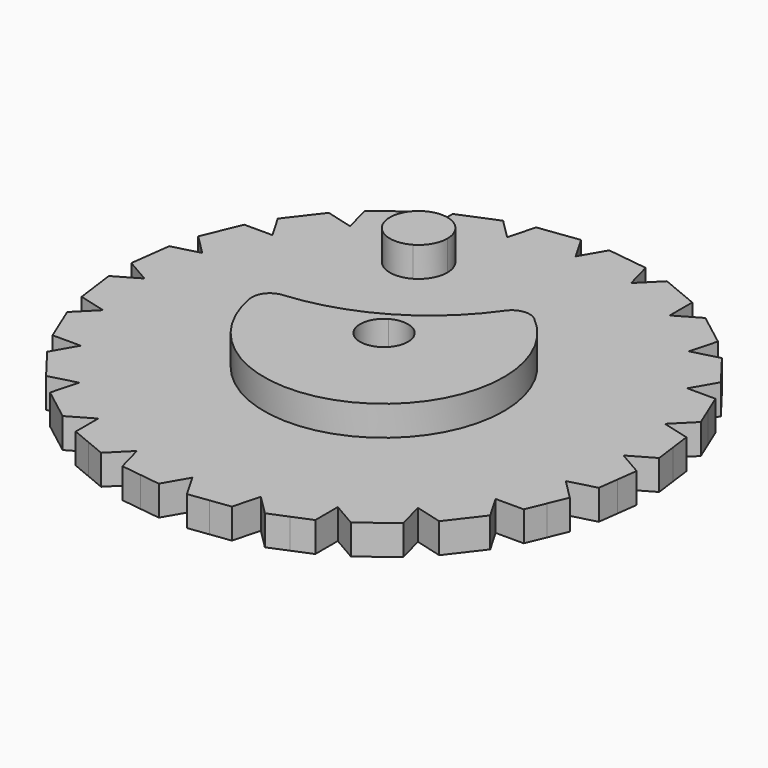
from build123d import *

# Parameters (mm, degrees)
F0_R     = 20
F2_DEPTH = 2.5
F3_DEPTH = 5
F4_DEPTH = 2.5
F5_R     = 1.5


with BuildPart() as f2:
    # F0 (on Top) → F2 (new body)
    with BuildSketch(Plane.XY):
        with Locations((30, 0)):
            Circle(F0_R)
        with BuildLine():
            ThreePointArc((20, 0), (24.4828773608, 0.5901820009), (28.6602540378, 2.3205080757))
            ThreePointArc((28.6602540378, 2.3205080757), (32.2474487139, 5.0730593618), (35, 8.6602540378))
            ThreePointArc((35, 8.6602540378), (35, -8.6602540378), (20, 0))
        make_face(mode=Mode.SUBTRACT)
        with BuildLine():
            ThreePointArc((24.9, 12.9903810568), (24.5784609691, 11.7903810568), (23.7, 10.9119200877))
            ThreePointArc((23.7, 10.9119200877), (20.4215390309, 14.1903810568), (24.9, 12.9903810568))
        make_face(mode=Mode.SUBTRACT)
    extrude(amount=F2_DEPTH)

    # F0 (on Top) → F3 (join)
    with BuildSketch(Plane.XY):
        with BuildLine():
            ThreePointArc((24.9, 12.9903810568), (20.4215390309, 14.1903810568), (23.7, 10.9119200877))
            ThreePointArc((23.7, 10.9119200877), (24.5784609691, 11.7903810568), (24.9, 12.9903810568))
        make_face()
        with BuildLine():
            ThreePointArc((35, 8.6602540378), (32.2474487139, 5.0730593618), (28.6602540378, 2.3205080757))
            ThreePointArc((28.6602540378, 2.3205080757), (24.4828773608, 0.5901820009), (20, 0))
            ThreePointArc((20, 0), (35, -8.6602540378), (35, 8.6602540378))
        make_face()
        with BuildLine():
            ThreePointArc((32, 0), (29, -1.7320508076), (29, 1.7320508076))
            ThreePointArc((29, 1.7320508076), (31, 1.7320508076), (32, 0))
        make_face(mode=Mode.SUBTRACT)
    extrude(amount=F3_DEPTH)

    # F1 (on Top) → F4 (join)
    with BuildSketch(Plane.XY):
        with BuildLine():
            Line((31.1749923535, 22.0351464548), (30, 20))
            ThreePointArc((30, 20), (32.6105238444, 19.8288972275), (35.1763809021, 19.3185165258))
            Line((35.1763809021, 19.3185165258), (34.5681601042, 21.5884274457))
            Line((34.5681601042, 21.5884274457), (32.8715762288, 21.8117869502))
            Line((32.8715762288, 21.8117869502), (31.1749923535, 22.0351464548))
        make_face()
        with BuildLine():
            Line((7.9648535452, 1.1749923535), (10, 0))
            Line((10, 0), (7.9648535452, -1.1749923535))
            Line((7.9648535452, -1.1749923535), (8.1882130498, -2.8715762288))
            Line((8.1882130498, -2.8715762288), (8.4115725543, -4.5681601042))
            Line((8.4115725543, -4.5681601042), (10.6814834742, -5.1763809021))
            Line((10.6814834742, -5.1763809021), (9.0197933522, -6.8380710241))
            Line((9.0197933522, -6.8380710241), (9.6746502848, -8.419035512))
            Line((9.6746502848, -8.419035512), (10.3295072173, -10))
            Line((10.3295072173, -10), (12.6794919243, -10))
            Line((12.6794919243, -10), (11.5044995708, -12.0351464548))
            Line((11.5044995708, -12.0351464548), (12.5462265136, -13.3927514382))
            Line((12.5462265136, -13.3927514382), (13.5879534564, -14.7503564216))
            Line((13.5879534564, -14.7503564216), (15.8578643763, -14.1421356237))
            Line((15.8578643763, -14.1421356237), (15.2496435784, -16.4120465436))
            Line((15.2496435784, -16.4120465436), (16.6072485618, -17.4537734864))
            Line((16.6072485618, -17.4537734864), (17.9648535452, -18.4955004292))
            Line((17.9648535452, -18.4955004292), (20, -17.3205080757))
            Line((20, -17.3205080757), (20, -19.6704927827))
            Line((20, -19.6704927827), (21.580964488, -20.3253497152))
            Line((21.580964488, -20.3253497152), (23.1619289759, -20.9802066478))
            Line((23.1619289759, -20.9802066478), (24.8236190979, -19.3185165258))
            Line((24.8236190979, -19.3185165258), (25.4318398958, -21.5884274457))
            Line((25.4318398958, -21.5884274457), (27.1284237712, -21.8117869502))
            Line((27.1284237712, -21.8117869502), (28.8250076465, -22.0351464548))
            Line((28.8250076465, -22.0351464548), (30, -20))
            Line((30, -20), (31.1749923535, -22.0351464548))
            Line((31.1749923535, -22.0351464548), (32.8715762288, -21.8117869502))
            Line((32.8715762288, -21.8117869502), (34.5681601042, -21.5884274457))
            Line((34.5681601042, -21.5884274457), (35.1763809021, -19.3185165258))
            Line((35.1763809021, -19.3185165258), (36.8380710241, -20.9802066478))
            Line((36.8380710241, -20.9802066478), (38.419035512, -20.3253497152))
            Line((38.419035512, -20.3253497152), (40, -19.6704927827))
            Line((40, -19.6704927827), (40, -17.3205080757))
            Line((40, -17.3205080757), (42.0351464548, -18.4955004292))
            Line((42.0351464548, -18.4955004292), (43.3927514382, -17.4537734864))
            Line((43.3927514382, -17.4537734864), (44.7503564216, -16.4120465436))
            Line((44.7503564216, -16.4120465436), (44.1421356237, -14.1421356237))
            Line((44.1421356237, -14.1421356237), (46.4120465436, -14.7503564216))
            Line((46.4120465436, -14.7503564216), (47.4537734864, -13.3927514382))
            Line((47.4537734864, -13.3927514382), (48.4955004292, -12.0351464548))
            Line((48.4955004292, -12.0351464548), (47.3205080757, -10))
            Line((47.3205080757, -10), (49.6704927827, -10))
            Line((49.6704927827, -10), (50.3253497152, -8.419035512))
            Line((50.3253497152, -8.419035512), (50.9802066478, -6.8380710241))
            Line((50.9802066478, -6.8380710241), (49.3185165258, -5.1763809021))
            Line((49.3185165258, -5.1763809021), (51.5884274457, -4.5681601042))
            Line((51.5884274457, -4.5681601042), (51.8117869502, -2.8715762288))
            Line((51.8117869502, -2.8715762288), (52.0351464548, -1.1749923535))
            Line((52.0351464548, -1.1749923535), (50, 0))
            Line((50, 0), (52.0351464548, 1.1749923535))
            Line((52.0351464548, 1.1749923535), (51.8117869502, 2.8715762288))
            Line((51.8117869502, 2.8715762288), (51.5884274457, 4.5681601042))
            Line((51.5884274457, 4.5681601042), (49.3185165258, 5.1763809021))
            Line((49.3185165258, 5.1763809021), (50.9802066478, 6.8380710241))
            Line((50.9802066478, 6.8380710241), (50.3253497152, 8.419035512))
            Line((50.3253497152, 8.419035512), (49.6704927827, 10))
            Line((49.6704927827, 10), (47.3205080757, 10))
            Line((47.3205080757, 10), (48.4955004292, 12.0351464548))
            Line((48.4955004292, 12.0351464548), (47.4537734864, 13.3927514382))
            Line((47.4537734864, 13.3927514382), (46.4120465436, 14.7503564216))
            Line((46.4120465436, 14.7503564216), (44.1421356237, 14.1421356237))
            Line((44.1421356237, 14.1421356237), (44.7503564216, 16.4120465436))
            Line((44.7503564216, 16.4120465436), (43.3927514382, 17.4537734864))
            Line((43.3927514382, 17.4537734864), (42.0351464548, 18.4955004292))
            Line((42.0351464548, 18.4955004292), (40, 17.3205080757))
            Line((40, 17.3205080757), (40, 19.6704927827))
            Line((40, 19.6704927827), (38.419035512, 20.3253497152))
            Line((38.419035512, 20.3253497152), (36.8380710241, 20.9802066478))
            Line((36.8380710241, 20.9802066478), (35.1763809021, 19.3185165258))
            ThreePointArc((35.1763809021, 19.3185165258), (32.6105238444, 19.8288972275), (30, 20))
            Line((30, 20), (28.8250076465, 22.0351464548))
            Line((28.8250076465, 22.0351464548), (27.1284237712, 21.8117869502))
            Line((27.1284237712, 21.8117869502), (25.4318398958, 21.5884274457))
            Line((25.4318398958, 21.5884274457), (24.8236190979, 19.3185165258))
            Line((24.8236190979, 19.3185165258), (23.1619289759, 20.9802066478))
            Line((23.1619289759, 20.9802066478), (21.580964488, 20.3253497152))
            Line((21.580964488, 20.3253497152), (20, 19.6704927827))
            Line((20, 19.6704927827), (20, 17.3205080757))
            Line((20, 17.3205080757), (17.9648535452, 18.4955004292))
            Line((17.9648535452, 18.4955004292), (16.6072485618, 17.4537734864))
            Line((16.6072485618, 17.4537734864), (15.2496435784, 16.4120465436))
            Line((15.2496435784, 16.4120465436), (15.8578643763, 14.1421356237))
            Line((15.8578643763, 14.1421356237), (13.5879534564, 14.7503564216))
            Line((13.5879534564, 14.7503564216), (12.5462265136, 13.3927514382))
            Line((12.5462265136, 13.3927514382), (11.5044995708, 12.0351464548))
            Line((11.5044995708, 12.0351464548), (12.6794919243, 10))
            Line((12.6794919243, 10), (10.3295072173, 10))
            Line((10.3295072173, 10), (9.6746502848, 8.419035512))
            Line((9.6746502848, 8.419035512), (9.0197933522, 6.8380710241))
            Line((9.0197933522, 6.8380710241), (10.6814834742, 5.1763809021))
            Line((10.6814834742, 5.1763809021), (8.4115725543, 4.5681601042))
            Line((8.4115725543, 4.5681601042), (8.1882130498, 2.8715762288))
            Line((8.1882130498, 2.8715762288), (7.9648535452, 1.1749923535))
        make_face()
        with BuildLine():
            ThreePointArc((32, 0), (30, -2), (28, 0))
            ThreePointArc((28, 0), (30, 2), (32, 0))
        make_face(mode=Mode.SUBTRACT)
    extrude(amount=F4_DEPTH)

    # F5
    f5_edges = [f2.edges().sort_by_distance(p)[0] for p in [
        (20, 0, 3.75),
        (35, 8.660254, 3.75),
    ]]
    fillet(f5_edges, radius=F5_R)


solid = f2.part
